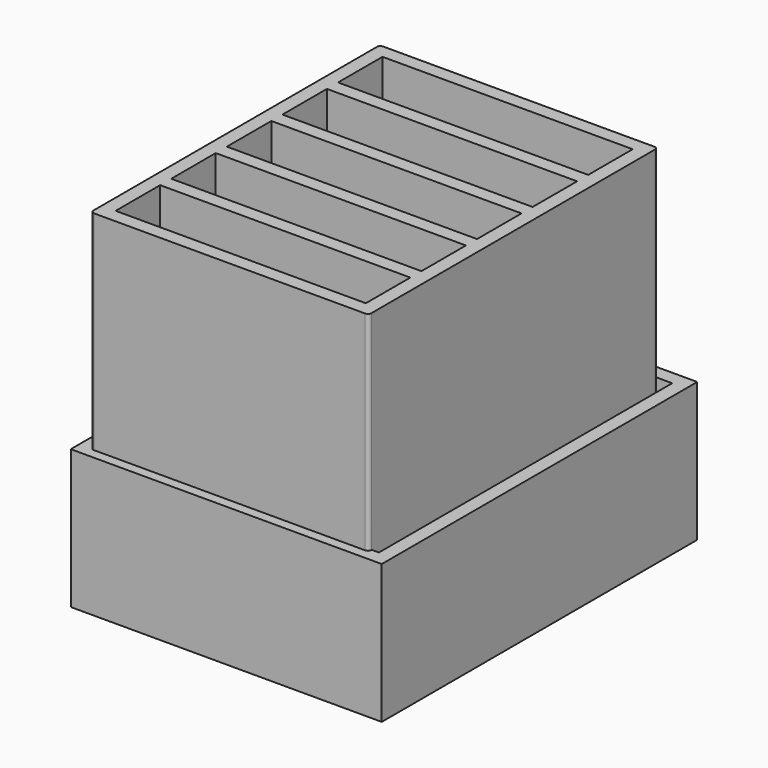
from build123d import *

# Parameters (mm, degrees)
F0_W     = 36
F0_H     = 8
F1_DEPTH = 2
F2_DEPTH = 50
F3_W     = 44.75
F3_H     = 56.75
F3_W_2   = 40.75
F3_H_2   = 52.75
F4_DEPTH = 2
F5_DEPTH = 20


with BuildPart() as f1:
    # F0 (on Top) → F1 (new body)
    with BuildSketch(Plane.XY):
        with BuildLine():
            Line((-23.2728253603, 79.1923393011), (-62.2728253603, 79.1923393011))
            ThreePointArc((-62.2728253603, 79.1923393011), (-62.6263787509, 79.0458926917), (-62.7728253603, 78.6923393011))
            Line((-62.7728253603, 78.6923393011), (-62.7728253603, 27.6923393011))
            ThreePointArc((-62.7728253603, 27.6923393011), (-62.6263787509, 27.3387859105), (-62.2728253603, 27.1923393011))
            Line((-62.2728253603, 27.1923393011), (-23.2728253603, 27.1923393011))
            ThreePointArc((-23.2728253603, 27.1923393011), (-22.9192719697, 27.3387859105), (-22.7728253603, 27.6923393011))
            Line((-22.7728253603, 27.6923393011), (-22.7728253603, 78.6923393011))
            ThreePointArc((-22.7728253603, 78.6923393011), (-22.9192719697, 79.0458926917), (-23.2728253603, 79.1923393011))
        make_face()
        with Locations((-42.7728253603, 33.1923393011)):
            Rectangle(F0_W, F0_H, mode=Mode.SUBTRACT)
        with Locations((-42.7728253603, 43.1923393011)):
            Rectangle(F0_W, F0_H, mode=Mode.SUBTRACT)
        with Locations((-42.7728253603, 53.1923393011)):
            Rectangle(F0_W, F0_H, mode=Mode.SUBTRACT)
        with Locations((-42.7728253603, 63.1923393011)):
            Rectangle(F0_W, F0_H, mode=Mode.SUBTRACT)
        with Locations((-42.7728253603, 73.1923393011)):
            Rectangle(F0_W, F0_H, mode=Mode.SUBTRACT)
        with Locations((-42.7728253603, 33.1923393011)):
            Rectangle(F0_W, F0_H)
        with Locations((-42.7728253603, 43.1923393011)):
            Rectangle(F0_W, F0_H)
        with Locations((-42.7728253603, 53.1923393011)):
            Rectangle(F0_W, F0_H)
        with Locations((-42.7728253603, 63.1923393011)):
            Rectangle(F0_W, F0_H)
        with Locations((-42.7728253603, 73.1923393011)):
            Rectangle(F0_W, F0_H)
    extrude(amount=F1_DEPTH)

    # F0 (on Top) → F2 (join)
    with BuildSketch(Plane.XY):
        with BuildLine():
            Line((-23.2728253603, 79.1923393011), (-62.2728253603, 79.1923393011))
            ThreePointArc((-62.2728253603, 79.1923393011), (-62.6263787509, 79.0458926917), (-62.7728253603, 78.6923393011))
            Line((-62.7728253603, 78.6923393011), (-62.7728253603, 27.6923393011))
            ThreePointArc((-62.7728253603, 27.6923393011), (-62.6263787509, 27.3387859105), (-62.2728253603, 27.1923393011))
            Line((-62.2728253603, 27.1923393011), (-23.2728253603, 27.1923393011))
            ThreePointArc((-23.2728253603, 27.1923393011), (-22.9192719697, 27.3387859105), (-22.7728253603, 27.6923393011))
            Line((-22.7728253603, 27.6923393011), (-22.7728253603, 78.6923393011))
            ThreePointArc((-22.7728253603, 78.6923393011), (-22.9192719697, 79.0458926917), (-23.2728253603, 79.1923393011))
        make_face()
        with Locations((-42.7728253603, 33.1923393011)):
            Rectangle(F0_W, F0_H, mode=Mode.SUBTRACT)
        with Locations((-42.7728253603, 43.1923393011)):
            Rectangle(F0_W, F0_H, mode=Mode.SUBTRACT)
        with Locations((-42.7728253603, 53.1923393011)):
            Rectangle(F0_W, F0_H, mode=Mode.SUBTRACT)
        with Locations((-42.7728253603, 63.1923393011)):
            Rectangle(F0_W, F0_H, mode=Mode.SUBTRACT)
        with Locations((-42.7728253603, 73.1923393011)):
            Rectangle(F0_W, F0_H, mode=Mode.SUBTRACT)
    extrude(amount=F2_DEPTH)


with BuildPart() as f4:
    # F3 (on Top) → F4 (new body)
    with BuildSketch(Plane.XY):
        with Locations((-42.1058821133, 54.1254512433)):
            Rectangle(F3_W, F3_H)
        with Locations((-42.1058821133, 54.1254512433)):
            Rectangle(F3_W_2, F3_H_2, mode=Mode.SUBTRACT)
        with Locations((-42.1058821133, 54.1254512433)):
            Rectangle(F3_W_2, F3_H_2)
    extrude(amount=F4_DEPTH)

    # F3 (on Top) → F5 (join)
    with BuildSketch(Plane.XY):
        with Locations((-42.1058821133, 54.1254512433)):
            Rectangle(F3_W, F3_H)
        with Locations((-42.1058821133, 54.1254512433)):
            Rectangle(F3_W_2, F3_H_2, mode=Mode.SUBTRACT)
    extrude(amount=F5_DEPTH)


solid = Compound([f1.part, f4.part])
